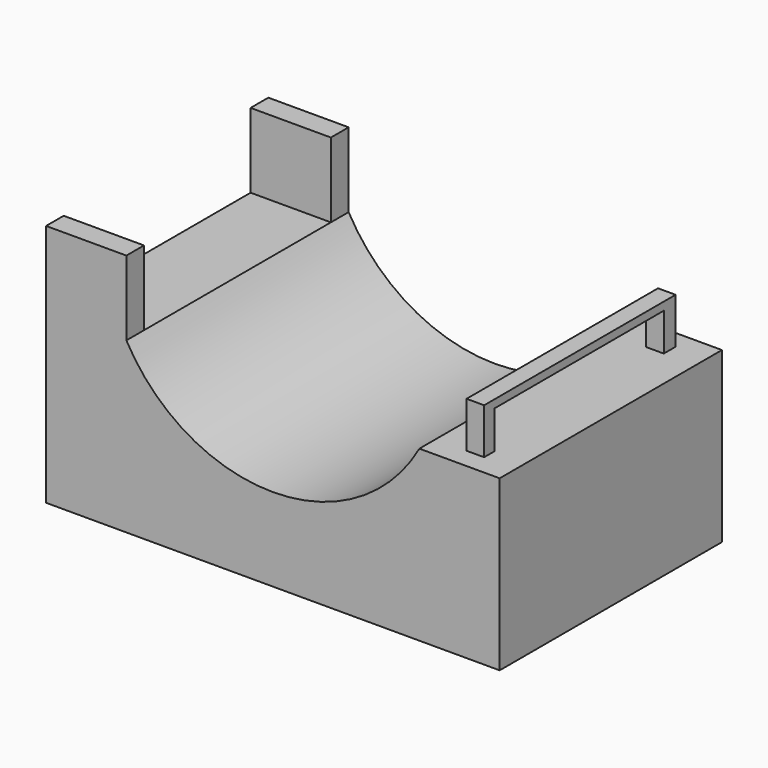
from build123d import *

# Parameters (mm, degrees)
F0_W      = 92.690166086
F0_H      = 53.4883048385
F1_DEPTH  = 87.884
F3_DEPTH  = 162.814
F4_DEPTH  = 25.4
F5_DEPTH  = 25.4
F6_W      = 5.5537819862
F6_H      = 75.7047273219
F7_DEPTH  = 14.478
F8_W      = 66.9379513711
F8_H      = 11.9429174811
F9_DEPTH  = 64.262
F10_W     = 133.9104250073
F10_H     = 74.4668878615
F11_DEPTH = 21.336
F12_DEPTH = 25.4
F13_W     = 25.4
F13_H     = 87.884
F14_DEPTH = 25.4
F15_W     = 25.4
F15_H     = 7.0143197663
F15_H_2   = 6.9646001425
F16_DEPTH = 42.418
F17_DEPTH = 18.796


with BuildPart() as f1:
    # F0 (on Front) → F1 (new body)
    with BuildSketch(Plane.XZ):
        with Locations((14.3755543977, -7.2218449786)):
            Rectangle(F0_W, F0_H)
    extrude(amount=F1_DEPTH)

    # F2 (on face) → F3 (cut)
    with BuildSketch(Plane.XZ.offset(87.884)):
        with BuildLine():
            Line((60.7206374407, 19.5223074406), (-31.9695286453, 19.5223074406))
            ThreePointArc((-31.9695286453, 19.5223074406), (14.3755543977, -7.6549383903), (60.7206374407, 19.5223074406))
        make_face()
    extrude(amount=-F3_DEPTH, mode=Mode.SUBTRACT)

    # F4 (add): a face of the model
    f4_faces = [f1.faces().sort_by_distance(p)[0] for p in [
        (60.7206374407, -43.942, -7.2218449786),
    ]]
    extrude(f4_faces, amount=F4_DEPTH)

    # F5 (add): a face of the model
    f5_faces = [f1.faces().sort_by_distance(p)[0] for p in [
        (-31.9695286453, -43.942, -7.2218449786),
    ]]
    extrude(f5_faces, amount=F5_DEPTH)

    # F6 (on face) → F7 (join)
    with BuildSketch(Plane.XY.offset(19.5223074406)):
        with Locations((73.3140408993, -43.6391439289)):
            Rectangle(F6_W, F6_H)
    extrude(amount=F7_DEPTH)

    # F8 (on face) → F9 (cut)
    with BuildSketch(Plane(origin=(70.5371499062, 0, 0), x_dir=(0, -1, 0), z_dir=(-1, 0, 0))):
        with Locations((43.9264485613, 25.4937661812)):
            Rectangle(F8_W, F8_H)
    extrude(amount=-F9_DEPTH, mode=Mode.SUBTRACT)

    # F10 (on face) → F11 (cut)
    with BuildSketch(Plane(origin=(0, 0, -33.9659973979), x_dir=(1, 0, 0), z_dir=(0, 0, -1))):
        with Locations((14.4990645349, 43.2672258466)):
            Rectangle(F10_W, F10_H)
    extrude(amount=-F11_DEPTH, mode=Mode.SUBTRACT)

    # F12 (add): a face of the model
    f12_faces = [f1.faces().sort_by_distance(p)[0] for p in [
        (-44.6695286453, -43.942, 19.5223074406),
    ]]
    extrude(f12_faces, amount=F12_DEPTH)

    # F13 (on face) → F14 (cut)
    with BuildSketch(Plane.XY.offset(44.9223074406)):
        with Locations((-44.6695286453, -43.942)):
            Rectangle(F13_W, F13_H)
    extrude(amount=-F14_DEPTH, mode=Mode.SUBTRACT)

    # F15 (on face) → F16 (join)
    with BuildSketch(Plane.XY.offset(19.5223074406)):
        with Locations((-44.6695286453, -3.5071598832)):
            Rectangle(F15_W, F15_H)
        with Locations((-44.6695286453, -84.4016999288)):
            Rectangle(F15_W, F15_H_2)
    extrude(amount=F16_DEPTH)

    # F17 (cut): faces of the model
    f17_faces = [f1.faces().sort_by_distance(p)[0] for p in [
        (-44.6695286453, -84.4016999288, 61.9403074406),
        (-44.6695286453, -3.5071598832, 61.9403074406),
    ]]
    extrude(f17_faces, amount=-F17_DEPTH, mode=Mode.SUBTRACT)


solid = f1.part
